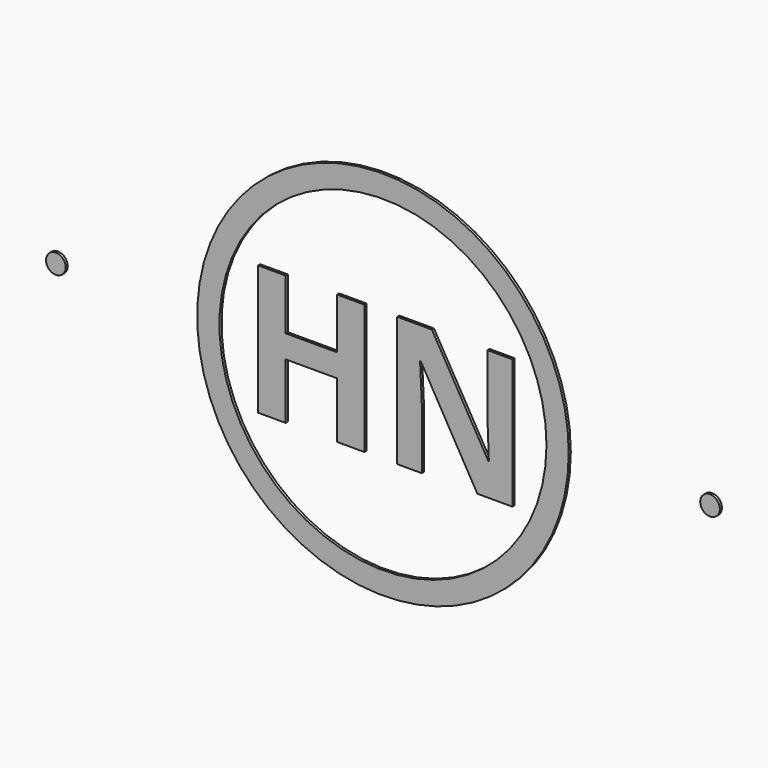
from build123d import *

# Parameters (mm, degrees)
F0_R          = 17.5
F1_DEPTH      = 1
F2_R          = 17.5
F2_R_2        = 15.25
F3_DEPTH      = 1
F4_R          = 17.5
F5_DEPTH      = 1
F6_R          = 14.2
F6_R_2        = 12.5
F6_TEXT_SIZE  = 13.8888888889
F7_DEPTH      = 0.2
F8_R          = 16.5
F8_R_2        = 15
F8_TEXT_SIZE  = 9.0277777778
F9_DEPTH      = 0.2
F11_DEPTH     = 0.4
F15_R         = 4
F15_R_2       = 2
F16_DEPTH     = 3
F17_T1_DEPTH  = 2
F17_T3_DEPTH  = 1
F18_F1_R      = 1.5
F18_F2_R      = 1.5
F19_R         = 0.75
F20_DEPTH     = 0.2
F21_R         = 14.2
F21_R_2       = 12.5
F21_TEXT_SIZE = 13.8888888889
F22_DEPTH     = 0.2


# Not quite as in the source:
# - a fillet or chamfer that OpenCascade refuses, or shapes differently, is made with other operations: its cross-section is extruded or revolved along the edge and cut away or added
# - a feature of the source that left no trace in its solid (it failed there, or was rolled back) is left out
# - a feature names something its author has since deleted; it is built from what else it names
# - Text() gives the source's letters only with a copy of the font that has no kerning and outlines rounded to 1/6400 em; it was checked with that copy


with BuildPart() as f1:
    # F0 (on Front) → F1 (new body)
    with BuildSketch(Plane.XZ):
        Circle(F0_R)
    extrude(amount=F1_DEPTH)

    # F2 (on face) → F3 (join)
    with BuildSketch(Plane(origin=(0, 0, 0), x_dir=(-1, 0, 0), z_dir=(0, 1, 0))):
        Circle(F2_R)
        Circle(F2_R_2, mode=Mode.SUBTRACT)
    extrude(amount=F3_DEPTH)

    # F4 (on face) → F5 (join)
    with BuildSketch(Plane(origin=(0, 1, 0), x_dir=(-1, 0, 0), z_dir=(0, 1, 0))):
        Circle(F4_R)
    extrude(amount=F5_DEPTH)

    # F6 (on face) → F7 (cut)
    with BuildSketch(Plane.XZ.offset(1)):
        Circle(F6_R)
        Circle(F6_R_2, mode=Mode.SUBTRACT)
        with Locations((-10.7855902778, -5)):
            Text('HN', F6_TEXT_SIZE, font='Open Sans', font_style=FontStyle.BOLD, text_align=(TextAlign.LEFT, TextAlign.BOTTOM))
    extrude(amount=-F7_DEPTH, mode=Mode.SUBTRACT)

    # F10 (on face) → F11 (join)
    with BuildSketch(Plane(origin=(0, 2, 0), x_dir=(-1, 0, 0), z_dir=(0, 1, 0))):
        with BuildLine():
            Line((-4.7, 4), (12.6279654253, -6.4941888806))
            ThreePointArc((12.6279654253, -6.4941888806), (14.1903368347, -0.5237752562), (13.0723614134, 5.545571844))
            Line((13.0723614134, 5.545571844), (2.6, 0.1635091373))
            Line((2.6, 0.1635091373), (12.3054412158, 7.0863330774))
            ThreePointArc((12.3054412158, 7.0863330774), (12.1529834417, 7.3447255541), (11.9951006995, 7.59983942))
            Line((11.9951006995, 7.59983942), (0.9, 1.1930657331))
            Line((0.9, 1.1930657331), (11.2941299736, 8.6071265901))
            ThreePointArc((11.2941299736, 8.6071265901), (11.1097684786, 8.843813903), (10.920447696, 9.0765534273))
            Line((10.920447696, 9.0765534273), (-0.8, 2.222622329))
            Line((-0.8, 2.222622329), (10.0907007992, 9.9908837137))
            ThreePointArc((10.0907007992, 9.9908837137), (9.8773735981, 10.2018376189), (9.6596372379, 10.4082375277))
            Line((9.6596372379, 10.4082375277), (-2.5, 3.2521789249))
            Line((-2.5, 3.2521789249), (8.6876874226, 11.2322788092))
            ThreePointArc((8.6876874226, 11.2322788092), (8.4484467099, 11.4133145137), (8.2054346966, 11.5892554308))
            Line((8.2054346966, 11.5892554308), (-4.2, 4.2817355208))
            Line((-4.2, 4.2817355208), (7.0655593046, 12.3173808788))
            ThreePointArc((7.0655593046, 12.3173808788), (-14.1981114568, -0.231583809), (7.4635087632, -12.0803988735))
            Line((7.4635087632, -12.0803988735), (-4.7, -5.9))
            Line((-4.7, -5.9), (-4.7, -4.4))
            Line((-4.7, -4.4), (7.7170485866, -11.9200319258))
            ThreePointArc((7.7170485866, -11.9200319258), (8.3915080931, -11.4552429884), (9.0380462181, -10.9523385886))
            Line((9.0380462181, -10.9523385886), (-4.7, -3.8))
            Line((-4.7, -3.8), (-4.7, -2.3))
            Line((-4.7, -2.3), (9.2674037222, -10.7589603703))
            ThreePointArc((9.2674037222, -10.7589603703), (9.8423672704, -10.2356146134), (10.3878254934, -9.6815846594))
            Line((10.3878254934, -9.6815846594), (-4.7, -1.7))
            Line((-4.7, -1.7), (-4.7, -0.2))
            Line((-4.7, -0.2), (10.5900363512, -9.4599751628))
            ThreePointArc((10.5900363512, -9.4599751628), (11.0780217671, -8.8835484874), (11.5346697714, -8.2819921073))
            Line((11.5346697714, -8.2819921073), (-4.7, 0.4))
            Line((-4.7, 0.4), (-4.7, 1.9))
            Line((-4.7, 1.9), (11.7070574809, -8.0364672051))
            ThreePointArc((11.7070574809, -8.0364672051), (12.114342533, -7.4082862386), (12.4879537237, -6.7595126892))
            Line((12.4879537237, -6.7595126892), (-4.7, 2.5))
            Line((-4.7, 2.5), (-4.7, 4))
        make_face()
    extrude(amount=F11_DEPTH)

    # F15 (on face) → F16 (join, through all)
    with BuildSketch(Plane.XZ.offset(1)):
        with Locations((0, 19.5)):
            Circle(F15_R)
        with Locations((0, 19.5)):
            Circle(F15_R_2, mode=Mode.SUBTRACT)
    extrude(amount=-F16_DEPTH)

    # F17: fillet of radius 5 on 4 edges, made by hand

    # F17_s2 → F17_t1 (join)
    with BuildSketch(Plane.XZ.offset(-2)):
        with BuildLine():
            ThreePointArc((6.9421534249, 16.0640283191), (4.9322938144, 17.6449218459), (3.9668947545, 20.0127826214))
            Line((3.9668947545, 20.0127826214), (3.8677199063, 19.9999627354))
            ThreePointArc((3.8677199063, 19.9999627354), (3.785225744, 18.5608162764), (3.1855140872, 17.25))
            Line((3.1855140872, 17.25), (3.248524256, 17.0940659341))
            ThreePointArc((3.248524256, 17.0940659341), (5.1064140249, 16.633837074), (6.90248375, 15.972233347))
            Line((6.90248375, 15.972233347), (6.9421534249, 16.0640283191))
        make_face()
        with BuildLine():
            ThreePointArc((-6.9421534249, 16.0640283191), (-4.9322938144, 17.6449218459), (-3.9668947545, 20.0127826214))
            Line((-3.9668947545, 20.0127826214), (-3.8677199063, 19.9999627354))
            ThreePointArc((-3.8677199063, 19.9999627354), (-3.785225744, 18.5608162764), (-3.1855140872, 17.25))
            Line((-3.1855140872, 17.25), (-3.248524256, 17.0940659341))
            ThreePointArc((-3.248524256, 17.0940659341), (-5.1064140249, 16.633837074), (-6.90248375, 15.972233347))
            Line((-6.90248375, 15.972233347), (-6.9421534249, 16.0640283191))
        make_face()
    extrude(amount=F17_T1_DEPTH)

    # F17_s4 → F17_t3 (join)
    with BuildSketch(Plane.XZ):
        with BuildLine():
            ThreePointArc((-6.9421534249, 16.0640283191), (-4.9322938144, 17.6449218459), (-3.9668947545, 20.0127826214))
            Line((-3.9668947545, 20.0127826214), (-3.8677199063, 19.9999627354))
            ThreePointArc((-3.8677199063, 19.9999627354), (-3.785225744, 18.5608162764), (-3.1855140872, 17.25))
            Line((-3.1855140872, 17.25), (-3.248524256, 17.0940659341))
            ThreePointArc((-3.248524256, 17.0940659341), (-5.1064140249, 16.633837074), (-6.90248375, 15.972233347))
            Line((-6.90248375, 15.972233347), (-6.9421534249, 16.0640283191))
        make_face()
        with BuildLine():
            ThreePointArc((3.9668947545, 20.0127826214), (4.9322938144, 17.6449218459), (6.9421534249, 16.0640283191))
            Line((6.9421534249, 16.0640283191), (6.90248375, 15.972233347))
            ThreePointArc((6.90248375, 15.972233347), (5.1064140249, 16.633837074), (3.248524256, 17.0940659341))
            Line((3.248524256, 17.0940659341), (3.1855140872, 17.25))
            ThreePointArc((3.1855140872, 17.25), (3.785225744, 18.5608162764), (3.8677199063, 19.9999627354))
            Line((3.8677199063, 19.9999627354), (3.9668947545, 20.0127826214))
        make_face()
    extrude(amount=F17_T3_DEPTH)

    # F18: fillet of radius 1.5 on 3 edges, made by hand

    # F18_f1
    f18_f1_edges = [f1.edges().sort_by_distance(p)[0] for p in [
        (-4.9302466516, -1, 17.647640759),
        (0, -1, -17.5),
        (4.9302466516, -1, 17.647640759),
        (0, -1, 23.5),
    ]]
    fillet(f18_f1_edges, radius=F18_F1_R)

    # F18_f2
    f18_f2_edges = [f1.edges().sort_by_distance(p)[0] for p in [
        (-2, 2, 19.5),
    ]]
    fillet(f18_f2_edges, radius=F18_F2_R)

    # F18_s3 → F18_t4 (revolve, cut)
    with BuildSketch(Plane.XY.offset(19.5)):
        with BuildLine():
            ThreePointArc((2, 0.5), (2.4393398282, -0.5606601718), (3.5, -1))
            Line((3.5, -1), (3.5, -1.03))
            Line((3.5, -1.03), (1.97, -1.03))
            Line((1.97, -1.03), (1.97, 0.5))
            Line((1.97, 0.5), (2, 0.5))
        make_face()
    revolve(axis=Axis((0, -1, 19.5), (0, 1, 0)), mode=Mode.SUBTRACT)


with BuildPart() as f9:
    # F8 (on face) → F9 (new body)
    with BuildSketch(Plane.XZ.offset(0.8)):
        Circle(F8_R)
        Circle(F8_R_2, mode=Mode.SUBTRACT)
        with BuildLine():
            Line((4.5413953993, -9), (6.2778320313, -9))
            Line((6.2778320313, -9), (6.2778320313, -2.5550130208))
            Line((6.2778320313, -2.5550130208), (5.047797309, -2.5550130208))
            Line((5.047797309, -2.5550130208), (5.047797309, -5.6061197917))
            add(Edge.make_bspline(
                [(5.1140950521, -7.3820529514), (5.047797309, -6.1252170139), (5.047797309, -5.6061197917)],
                knots=[0, 0, 0, 1, 1, 1], degree=2))
            Line((5.1140950521, -7.3820529514), (5.083062066, -7.3820529514))
            Line((5.083062066, -7.3820529514), (2.2844509549, -2.5550130208))
            Line((2.2844509549, -2.5550130208), (0.5607096354, -2.5550130208))
            Line((0.5607096354, -2.5550130208), (0.5607096354, -9))
            Line((0.5607096354, -9), (1.782280816, -9))
            Line((1.782280816, -9), (1.782280816, -5.9672309028))
            add(Edge.make_bspline(
                [(1.6976453993, -4.125), (1.782280816, -5.4156901042), (1.782280816, -5.9672309028)],
                knots=[0, 0, 0, 1, 1, 1], degree=2))
            Line((1.6976453993, -4.125), (1.7371419271, -4.125))
            Line((1.7371419271, -4.125), (4.5413953993, -9))
        make_face()
        with BuildLine():
            Line((-5.0026584201, -9), (-3.6400282118, -9))
            Line((-3.6400282118, -9), (-3.6400282118, -2.5550130208))
            Line((-3.6400282118, -2.5550130208), (-5.0026584201, -2.5550130208))
            Line((-5.0026584201, -2.5550130208), (-5.0026584201, -5.0813802083))
            Line((-5.0026584201, -5.0813802083), (-7.5544162326, -5.0813802083))
            Line((-7.5544162326, -5.0813802083), (-7.5544162326, -2.5550130208))
            Line((-7.5544162326, -2.5550130208), (-8.9212782118, -2.5550130208))
            Line((-8.9212782118, -2.5550130208), (-8.9212782118, -8.7556150594))
            ThreePointArc((-8.9212782118, -8.7556150594), (-8.7988255055, -8.8786637352), (-8.6746757864, -9))
            Line((-8.6746757864, -9), (-7.5544162326, -9))
            Line((-7.5544162326, -9), (-7.5544162326, -6.2183159722))
            Line((-7.5544162326, -6.2183159722), (-5.0026584201, -6.2183159722))
            Line((-5.0026584201, -6.2183159722), (-5.0026584201, -9))
        make_face()
        with Locations((-7.3519965278, 2.5)):
            Text('VIP', F8_TEXT_SIZE, font='Open Sans', font_style=FontStyle.BOLD, text_align=(TextAlign.LEFT, TextAlign.BOTTOM))
        with BuildLine():
            add(Edge.make_bspline(
                [(-2.3084309896, -8.3694661458), (-2.3084309896, -7.9998914931), (-2.1102430556, -7.8101671007)],
                knots=[0, 0, 0, 1, 1, 1], degree=2))
            add(Edge.make_bspline(
                [(-2.1060112847, -8.9224175347), (-2.3084309896, -8.7263454861), (-2.3084309896, -8.3694661458)],
                knots=[0, 0, 0, 1, 1, 1], degree=2))
            add(Edge.make_bspline(
                [(-1.5326063368, -9.1184895833), (-1.9035915799, -9.1184895833), (-2.1060112847, -8.9224175347)],
                knots=[0, 0, 0, 1, 1, 1], degree=2))
            add(Edge.make_bspline(
                [(-0.9690755208, -8.9181857639), (-1.1714952257, -9.1184895833), (-1.5326063368, -9.1184895833)],
                knots=[0, 0, 0, 1, 1, 1], degree=2))
            add(Edge.make_bspline(
                [(-0.766655816, -8.3694661458), (-0.766655816, -8.7178819444), (-0.9690755208, -8.9181857639)],
                knots=[0, 0, 0, 1, 1, 1], degree=2))
            add(Edge.make_bspline(
                [(-0.9669596354, -7.8143988715), (-0.766655816, -8.0083550347), (-0.766655816, -8.3694661458)],
                knots=[0, 0, 0, 1, 1, 1], degree=2))
            add(Edge.make_bspline(
                [(-1.5326063368, -7.6204427083), (-1.1672634549, -7.6204427083), (-0.9669596354, -7.8143988715)],
                knots=[0, 0, 0, 1, 1, 1], degree=2))
            add(Edge.make_bspline(
                [(-2.1102430556, -7.8101671007), (-1.9120551215, -7.6204427083), (-1.5326063368, -7.6204427083)],
                knots=[0, 0, 0, 1, 1, 1], degree=2))
        make_face()
        with BuildLine():
            add(Edge.make_bspline(
                [(8.5658348615, -9.1036516369), (8.4793062061, -9.1184895833), (8.3810221354, -9.1184895833)],
                knots=[0.7278287274, 0.7278287274, 0.7278287274, 1, 1, 1], degree=2))
            ThreePointArc((8.5658348615, -9.1036516369), (8.8548052444, -8.8228353766), (9.1345744701, -8.5328511794))
            add(Edge.make_bspline(
                [(9.1469726563, -8.3694661458), (9.1469726563, -8.4556945844), (9.1345744701, -8.5328511794)],
                knots=[0, 0, 0, 0.2474871659, 0.2474871659, 0.2474871659], degree=2))
            add(Edge.make_bspline(
                [(8.9466688368, -7.8143988715), (9.1469726563, -8.0083550347), (9.1469726563, -8.3694661458)],
                knots=[0, 0, 0, 1, 1, 1], degree=2))
            add(Edge.make_bspline(
                [(8.3810221354, -7.6204427083), (8.7463650174, -7.6204427083), (8.9466688368, -7.8143988715)],
                knots=[0, 0, 0, 1, 1, 1], degree=2))
            add(Edge.make_bspline(
                [(7.8033854167, -7.8101671007), (8.0015733507, -7.6204427083), (8.3810221354, -7.6204427083)],
                knots=[0, 0, 0, 1, 1, 1], degree=2))
            add(Edge.make_bspline(
                [(7.6051974826, -8.3694661458), (7.6051974826, -7.9998914931), (7.8033854167, -7.8101671007)],
                knots=[0, 0, 0, 1, 1, 1], degree=2))
            add(Edge.make_bspline(
                [(7.8076171875, -8.9224175347), (7.6051974826, -8.7263454861), (7.6051974826, -8.3694661458)],
                knots=[0, 0, 0, 1, 1, 1], degree=2))
            add(Edge.make_bspline(
                [(8.3810221354, -9.1184895833), (8.0100368924, -9.1184895833), (7.8076171875, -8.9224175347)],
                knots=[0, 0, 0, 1, 1, 1], degree=2))
        make_face()
    extrude(amount=F9_DEPTH)


with BuildPart() as f20:
    # F19 (on face) → F20 (new body)
    with BuildSketch(Plane.XZ.offset(1)):
        with Locations((25, 0)):
            Circle(F19_R)
    extrude(amount=-F20_DEPTH)


with BuildPart() as f20b:
    # F19 (on face) → F20, piece 2 (new body)
    with BuildSketch(Plane.XZ.offset(1)):
        with Locations((-25, 0)):
            Circle(F19_R)
    extrude(amount=-F20_DEPTH)


with BuildPart() as f22:
    # F21 (on face) → F22 (new body)
    with BuildSketch(Plane.XZ.offset(1)):
        Circle(F21_R)
        Circle(F21_R_2, mode=Mode.SUBTRACT)
        with Locations((-10.7855902778, -5)):
            Text('HN', F21_TEXT_SIZE, font='Open Sans', font_style=FontStyle.BOLD, text_align=(TextAlign.LEFT, TextAlign.BOTTOM))
    extrude(amount=-F22_DEPTH)


solid = Compound([f20.part, f20b.part, f22.part])
